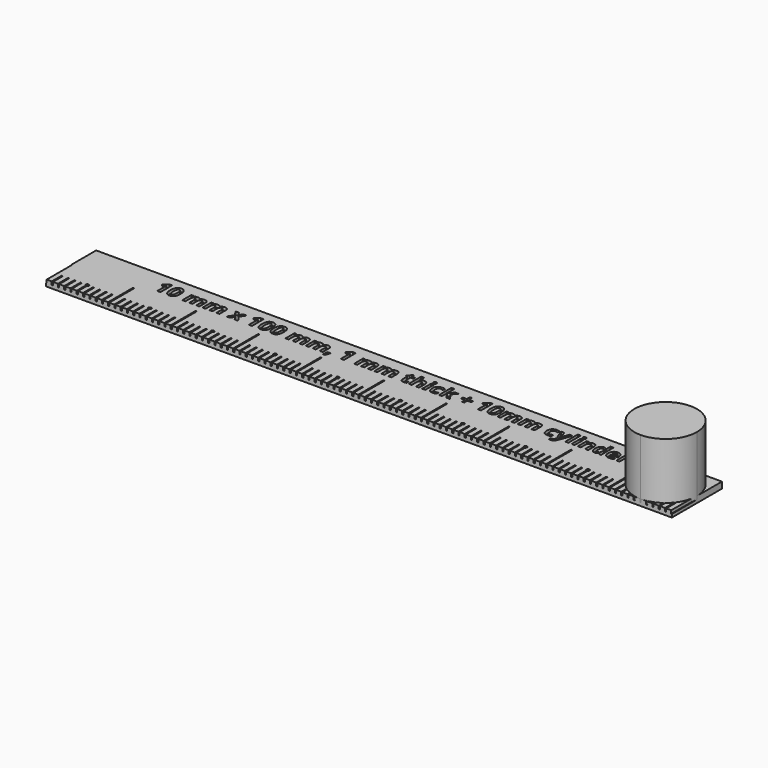
from build123d import *

# Parameters (mm, degrees)
F0_W         = 100
F0_H         = 10
F1_DEPTH     = 0.5
F3_DEPTH     = 0.5
F5_DEPTH     = 10
F6_TEXT_SIZE = 3.2776908483
F7_DEPTH     = 0.5


# Not quite as in the source:
# - Text() gives the source's letters only with a copy of the font that has no kerning and outlines rounded to 1/6400 em; it was checked with that copy


with BuildPart() as f1:
    # F0 (on Top) → F1 (new body)
    with BuildSketch(Plane.XY):
        Rectangle(F0_W, F0_H)
    extrude(amount=F1_DEPTH)

    # F2 (on face) → F3 (join)
    with BuildSketch(Plane.XY.offset(0.5)):
        with BuildLine():
            Line((-49.9, -0.1), (-49.9, -5))
            Line((-49.9, -5), (-49.1, -5))
            Line((-49.1, -5), (-49.1, -3))
            Line((-49.1, -3), (-48.9, -3))
            Line((-48.9, -3), (-48.9, -5))
            Line((-48.9, -5), (-48.1, -5))
            Line((-48.1, -5), (-48.1, -3))
            Line((-48.1, -3), (-47.9, -3))
            Line((-47.9, -3), (-47.9, -5))
            Line((-47.9, -5), (-47.1, -5))
            Line((-47.1, -5), (-47.1, -3))
            Line((-47.1, -3), (-46.9, -3))
            Line((-46.9, -3), (-46.9, -5))
            Line((-46.9, -5), (-46.1, -5))
            Line((-46.1, -5), (-46.1, -3))
            Line((-46.1, -3), (-45.9, -3))
            Line((-45.9, -3), (-45.9, -5))
            Line((-45.9, -5), (-45.1, -5))
            Line((-45.1, -5), (-45.1, -3.2291287847))
            ThreePointArc((-45.1, -3.2291287847), (-45.1369306394, -2.7908349934), (-44.75, -3))
            ThreePointArc((-44.75, -3), (-44.7908349934, -3.1369306394), (-44.9, -3.2291287847))
            Line((-44.9, -3.2291287847), (-44.9, -5))
            Line((-44.9, -5), (-44.1, -5))
            Line((-44.1, -5), (-44.1, -3))
            Line((-44.1, -3), (-43.9, -3))
            Line((-43.9, -3), (-43.9, -5))
            Line((-43.9, -5), (-43.1, -5))
            Line((-43.1, -5), (-43.1, -3))
            Line((-43.1, -3), (-42.9, -3))
            Line((-42.9, -3), (-42.9, -5))
            Line((-42.9, -5), (-42.1, -5))
            Line((-42.1, -5), (-42.1, -3))
            Line((-42.1, -3), (-41.9, -3))
            Line((-41.9, -3), (-41.9, -5))
            Line((-41.9, -5), (-41.1, -5))
            Line((-41.1, -5), (-41.1, -3))
            Line((-41.1, -3), (-40.9, -3))
            Line((-40.9, -3), (-40.9, -5))
            Line((-40.9, -5), (-40.1, -5))
            Line((-40.1, -5), (-40.1, -0.1))
            ThreePointArc((-40.1, -0.1), (-40, 0), (-39.9, -0.1))
            Line((-39.9, -0.1), (-39.9, -5))
            Line((-39.9, -5), (-39.1, -5))
            Line((-39.1, -5), (-39.1, -3))
            Line((-39.1, -3), (-38.9, -3))
            Line((-38.9, -3), (-38.9, -5))
            Line((-38.9, -5), (-38.1, -5))
            Line((-38.1, -5), (-38.1, -3))
            Line((-38.1, -3), (-37.9, -3))
            Line((-37.9, -3), (-37.9, -5))
            Line((-37.9, -5), (-37.1, -5))
            Line((-37.1, -5), (-37.1, -3))
            Line((-37.1, -3), (-36.9, -3))
            Line((-36.9, -3), (-36.9, -5))
            Line((-36.9, -5), (-36.1, -5))
            Line((-36.1, -5), (-36.1, -3))
            Line((-36.1, -3), (-35.9, -3))
            Line((-35.9, -3), (-35.9, -5))
            Line((-35.9, -5), (-35.1, -5))
            Line((-35.1, -5), (-35.1, -3.2291287847))
            ThreePointArc((-35.1, -3.2291287847), (-35.1369306394, -2.7908349934), (-34.75, -3))
            ThreePointArc((-34.75, -3), (-34.7908349934, -3.1369306394), (-34.9, -3.2291287847))
            Line((-34.9, -3.2291287847), (-34.9, -5))
            Line((-34.9, -5), (-34.1, -5))
            Line((-34.1, -5), (-34.1, -3))
            Line((-34.1, -3), (-33.9, -3))
            Line((-33.9, -3), (-33.9, -5))
            Line((-33.9, -5), (-33.1, -5))
            Line((-33.1, -5), (-33.1, -3))
            Line((-33.1, -3), (-32.9, -3))
            Line((-32.9, -3), (-32.9, -5))
            Line((-32.9, -5), (-32.1, -5))
            Line((-32.1, -5), (-32.1, -3))
            Line((-32.1, -3), (-31.9, -3))
            Line((-31.9, -3), (-31.9, -5))
            Line((-31.9, -5), (-31.1, -5))
            Line((-31.1, -5), (-31.1, -3))
            Line((-31.1, -3), (-30.9, -3))
            Line((-30.9, -3), (-30.9, -5))
            Line((-30.9, -5), (-30.1, -5))
            Line((-30.1, -5), (-30.1, -0.1))
            ThreePointArc((-30.1, -0.1), (-30, 0), (-29.9, -0.1))
            Line((-29.9, -0.1), (-29.9, -5))
            Line((-29.9, -5), (-29.1, -5))
            Line((-29.1, -5), (-29.1, -3))
            Line((-29.1, -3), (-28.9, -3))
            Line((-28.9, -3), (-28.9, -5))
            Line((-28.9, -5), (-28.1, -5))
            Line((-28.1, -5), (-28.1, -3))
            Line((-28.1, -3), (-27.9, -3))
            Line((-27.9, -3), (-27.9, -5))
            Line((-27.9, -5), (-27.1, -5))
            Line((-27.1, -5), (-27.1, -3))
            Line((-27.1, -3), (-26.9, -3))
            Line((-26.9, -3), (-26.9, -5))
            Line((-26.9, -5), (-26.1, -5))
            Line((-26.1, -5), (-26.1, -3))
            Line((-26.1, -3), (-25.9, -3))
            Line((-25.9, -3), (-25.9, -5))
            Line((-25.9, -5), (-25.1, -5))
            Line((-25.1, -5), (-25.1, -3.2291287847))
            ThreePointArc((-25.1, -3.2291287847), (-25.1369306394, -2.7908349934), (-24.75, -3))
            ThreePointArc((-24.75, -3), (-24.7908349934, -3.1369306394), (-24.9, -3.2291287847))
            Line((-24.9, -3.2291287847), (-24.9, -5))
            Line((-24.9, -5), (-24.1, -5))
            Line((-24.1, -5), (-24.1, -3))
            Line((-24.1, -3), (-23.9, -3))
            Line((-23.9, -3), (-23.9, -5))
            Line((-23.9, -5), (-23.1, -5))
            Line((-23.1, -5), (-23.1, -3))
            Line((-23.1, -3), (-22.9, -3))
            Line((-22.9, -3), (-22.9, -5))
            Line((-22.9, -5), (-22.1, -5))
            Line((-22.1, -5), (-22.1, -3))
            Line((-22.1, -3), (-21.9, -3))
            Line((-21.9, -3), (-21.9, -5))
            Line((-21.9, -5), (-21.1, -5))
            Line((-21.1, -5), (-21.1, -3))
            Line((-21.1, -3), (-20.9, -3))
            Line((-20.9, -3), (-20.9, -5))
            Line((-20.9, -5), (-20.1, -5))
            Line((-20.1, -5), (-20.1, -0.1))
            ThreePointArc((-20.1, -0.1), (-20, 0), (-19.9, -0.1))
            Line((-19.9, -0.1), (-19.9, -5))
            Line((-19.9, -5), (-19.1, -5))
            Line((-19.1, -5), (-19.1, -3))
            Line((-19.1, -3), (-18.9, -3))
            Line((-18.9, -3), (-18.9, -5))
            Line((-18.9, -5), (-18.1, -5))
            Line((-18.1, -5), (-18.1, -3))
            Line((-18.1, -3), (-17.9, -3))
            Line((-17.9, -3), (-17.9, -5))
            Line((-17.9, -5), (-17.1, -5))
            Line((-17.1, -5), (-17.1, -3))
            Line((-17.1, -3), (-16.9, -3))
            Line((-16.9, -3), (-16.9, -5))
            Line((-16.9, -5), (-16.1, -5))
            Line((-16.1, -5), (-16.1, -3))
            Line((-16.1, -3), (-15.9, -3))
            Line((-15.9, -3), (-15.9, -5))
            Line((-15.9, -5), (-15.1, -5))
            Line((-15.1, -5), (-15.1, -3.2291287847))
            ThreePointArc((-15.1, -3.2291287847), (-15.1369306394, -2.7908349934), (-14.75, -3))
            ThreePointArc((-14.75, -3), (-14.7908349934, -3.1369306394), (-14.9, -3.2291287847))
            Line((-14.9, -3.2291287847), (-14.9, -5))
            Line((-14.9, -5), (-14.1, -5))
            Line((-14.1, -5), (-14.1, -3))
            Line((-14.1, -3), (-13.9, -3))
            Line((-13.9, -3), (-13.9, -5))
            Line((-13.9, -5), (-13.1, -5))
            Line((-13.1, -5), (-13.1, -3))
            Line((-13.1, -3), (-12.9, -3))
            Line((-12.9, -3), (-12.9, -5))
            Line((-12.9, -5), (-12.1, -5))
            Line((-12.1, -5), (-12.1, -3))
            Line((-12.1, -3), (-11.9, -3))
            Line((-11.9, -3), (-11.9, -5))
            Line((-11.9, -5), (-11.1, -5))
            Line((-11.1, -5), (-11.1, -3))
            Line((-11.1, -3), (-10.9, -3))
            Line((-10.9, -3), (-10.9, -5))
            Line((-10.9, -5), (-10.1, -5))
            Line((-10.1, -5), (-10.1, -0.1))
            ThreePointArc((-10.1, -0.1), (-10, 0), (-9.9, -0.1))
            Line((-9.9, -0.1), (-9.9, -5))
            Line((-9.9, -5), (-9.1, -5))
            Line((-9.1, -5), (-9.1, -3))
            Line((-9.1, -3), (-8.9, -3))
            Line((-8.9, -3), (-8.9, -5))
            Line((-8.9, -5), (-8.1, -5))
            Line((-8.1, -5), (-8.1, -3))
            Line((-8.1, -3), (-7.9, -3))
            Line((-7.9, -3), (-7.9, -5))
            Line((-7.9, -5), (-7.1, -5))
            Line((-7.1, -5), (-7.1, -3))
            Line((-7.1, -3), (-6.9, -3))
            Line((-6.9, -3), (-6.9, -5))
            Line((-6.9, -5), (-6.1, -5))
            Line((-6.1, -5), (-6.1, -3))
            Line((-6.1, -3), (-5.9, -3))
            Line((-5.9, -3), (-5.9, -5))
            Line((-5.9, -5), (-5.1, -5))
            Line((-5.1, -5), (-5.1, -3.2291287847))
            ThreePointArc((-5.1, -3.2291287847), (-5.1369306394, -2.7908349934), (-4.75, -3))
            ThreePointArc((-4.75, -3), (-4.7908349934, -3.1369306394), (-4.9, -3.2291287847))
            Line((-4.9, -3.2291287847), (-4.9, -5))
            Line((-4.9, -5), (-4.1, -5))
            Line((-4.1, -5), (-4.1, -3))
            Line((-4.1, -3), (-3.9, -3))
            Line((-3.9, -3), (-3.9, -5))
            Line((-3.9, -5), (-3.1, -5))
            Line((-3.1, -5), (-3.1, -3))
            Line((-3.1, -3), (-2.9, -3))
            Line((-2.9, -3), (-2.9, -5))
            Line((-2.9, -5), (-2.1, -5))
            Line((-2.1, -5), (-2.1, -3))
            Line((-2.1, -3), (-1.9, -3))
            Line((-1.9, -3), (-1.9, -5))
            Line((-1.9, -5), (-1.1, -5))
            Line((-1.1, -5), (-1.1, -3))
            Line((-1.1, -3), (-0.9, -3))
            Line((-0.9, -3), (-0.9, -5))
            Line((-0.9, -5), (-0.1, -5))
            Line((-0.1, -5), (-0.1, -0.1))
            ThreePointArc((-0.1, -0.1), (0, 0), (0.1, -0.1))
            Line((0.1, -0.1), (0.1, -5))
            Line((0.1, -5), (0.9, -5))
            Line((0.9, -5), (0.9, -3))
            Line((0.9, -3), (1.1, -3))
            Line((1.1, -3), (1.1, -5))
            Line((1.1, -5), (1.9, -5))
            Line((1.9, -5), (1.9, -3))
            Line((1.9, -3), (2.1, -3))
            Line((2.1, -3), (2.1, -5))
            Line((2.1, -5), (2.9, -5))
            Line((2.9, -5), (2.9, -3))
            Line((2.9, -3), (3.1, -3))
            Line((3.1, -3), (3.1, -5))
            Line((3.1, -5), (3.9, -5))
            Line((3.9, -5), (3.9, -3))
            Line((3.9, -3), (4.1, -3))
            Line((4.1, -3), (4.1, -5))
            Line((4.1, -5), (4.9, -5))
            Line((4.9, -5), (4.9, -3.2291287847))
            ThreePointArc((4.9, -3.2291287847), (4.8630693606, -2.7908349934), (5.25, -3))
            ThreePointArc((5.25, -3), (5.2091650066, -3.1369306394), (5.1, -3.2291287847))
            Line((5.1, -3.2291287847), (5.1, -5))
            Line((5.1, -5), (5.9, -5))
            Line((5.9, -5), (5.9, -3))
            Line((5.9, -3), (6.1, -3))
            Line((6.1, -3), (6.1, -5))
            Line((6.1, -5), (6.9, -5))
            Line((6.9, -5), (6.9, -3))
            Line((6.9, -3), (7.1, -3))
            Line((7.1, -3), (7.1, -5))
            Line((7.1, -5), (7.9, -5))
            Line((7.9, -5), (7.9, -3))
            Line((7.9, -3), (8.1, -3))
            Line((8.1, -3), (8.1, -5))
            Line((8.1, -5), (8.9, -5))
            Line((8.9, -5), (8.9, -3))
            Line((8.9, -3), (9.1, -3))
            Line((9.1, -3), (9.1, -5))
            Line((9.1, -5), (9.9, -5))
            Line((9.9, -5), (9.9, -0.1))
            ThreePointArc((9.9, -0.1), (10, 0), (10.1, -0.1))
            Line((10.1, -0.1), (10.1, -5))
            Line((10.1, -5), (10.9, -5))
            Line((10.9, -5), (10.9, -3))
            Line((10.9, -3), (11.1, -3))
            Line((11.1, -3), (11.1, -5))
            Line((11.1, -5), (11.9, -5))
            Line((11.9, -5), (11.9, -3))
            Line((11.9, -3), (12.1, -3))
            Line((12.1, -3), (12.1, -5))
            Line((12.1, -5), (12.9, -5))
            Line((12.9, -5), (12.9, -3))
            Line((12.9, -3), (13.1, -3))
            Line((13.1, -3), (13.1, -5))
            Line((13.1, -5), (13.9, -5))
            Line((13.9, -5), (13.9, -3))
            Line((13.9, -3), (14.1, -3))
            Line((14.1, -3), (14.1, -5))
            Line((14.1, -5), (14.9, -5))
            Line((14.9, -5), (14.9, -3.2291287847))
            ThreePointArc((14.9, -3.2291287847), (14.8630693606, -2.7908349934), (15.25, -3))
            ThreePointArc((15.25, -3), (15.2091650066, -3.1369306394), (15.1, -3.2291287847))
            Line((15.1, -3.2291287847), (15.1, -5))
            Line((15.1, -5), (15.9, -5))
            Line((15.9, -5), (15.9, -3))
            Line((15.9, -3), (16.1, -3))
            Line((16.1, -3), (16.1, -5))
            Line((16.1, -5), (16.9, -5))
            Line((16.9, -5), (16.9, -3))
            Line((16.9, -3), (17.1, -3))
            Line((17.1, -3), (17.1, -5))
            Line((17.1, -5), (17.9, -5))
            Line((17.9, -5), (17.9, -3))
            Line((17.9, -3), (18.1, -3))
            Line((18.1, -3), (18.1, -5))
            Line((18.1, -5), (18.9, -5))
            Line((18.9, -5), (18.9, -3))
            Line((18.9, -3), (19.1, -3))
            Line((19.1, -3), (19.1, -5))
            Line((19.1, -5), (19.9, -5))
            Line((19.9, -5), (19.9, -0.1))
            ThreePointArc((19.9, -0.1), (20, 0), (20.1, -0.1))
            Line((20.1, -0.1), (20.1, -5))
            Line((20.1, -5), (20.9, -5))
            Line((20.9, -5), (20.9, -3))
            Line((20.9, -3), (21.1, -3))
            Line((21.1, -3), (21.1, -5))
            Line((21.1, -5), (21.9, -5))
            Line((21.9, -5), (21.9, -3))
            Line((21.9, -3), (22.1, -3))
            Line((22.1, -3), (22.1, -5))
            Line((22.1, -5), (22.9, -5))
            Line((22.9, -5), (22.9, -3))
            Line((22.9, -3), (23.1, -3))
            Line((23.1, -3), (23.1, -5))
            Line((23.1, -5), (23.9, -5))
            Line((23.9, -5), (23.9, -3))
            Line((23.9, -3), (24.1, -3))
            Line((24.1, -3), (24.1, -5))
            Line((24.1, -5), (24.9, -5))
            Line((24.9, -5), (24.9, -3.2291287847))
            ThreePointArc((24.9, -3.2291287847), (24.8630693606, -2.7908349934), (25.25, -3))
            ThreePointArc((25.25, -3), (25.2091650066, -3.1369306394), (25.1, -3.2291287847))
            Line((25.1, -3.2291287847), (25.1, -5))
            Line((25.1, -5), (25.9, -5))
            Line((25.9, -5), (25.9, -3))
            Line((25.9, -3), (26.1, -3))
            Line((26.1, -3), (26.1, -5))
            Line((26.1, -5), (26.9, -5))
            Line((26.9, -5), (26.9, -3))
            Line((26.9, -3), (27.1, -3))
            Line((27.1, -3), (27.1, -5))
            Line((27.1, -5), (27.9, -5))
            Line((27.9, -5), (27.9, -3))
            Line((27.9, -3), (28.1, -3))
            Line((28.1, -3), (28.1, -5))
            Line((28.1, -5), (28.9, -5))
            Line((28.9, -5), (28.9, -3))
            Line((28.9, -3), (29.1, -3))
            Line((29.1, -3), (29.1, -5))
            Line((29.1, -5), (29.9, -5))
            Line((29.9, -5), (29.9, -0.1))
            ThreePointArc((29.9, -0.1), (30, 0), (30.1, -0.1))
            Line((30.1, -0.1), (30.1, -5))
            Line((30.1, -5), (30.9, -5))
            Line((30.9, -5), (30.9, -3))
            Line((30.9, -3), (31.1, -3))
            Line((31.1, -3), (31.1, -5))
            Line((31.1, -5), (31.9, -5))
            Line((31.9, -5), (31.9, -3))
            Line((31.9, -3), (32.1, -3))
            Line((32.1, -3), (32.1, -5))
            Line((32.1, -5), (32.9, -5))
            Line((32.9, -5), (32.9, -3))
            Line((32.9, -3), (33.1, -3))
            Line((33.1, -3), (33.1, -5))
            Line((33.1, -5), (33.9, -5))
            Line((33.9, -5), (33.9, -3))
            Line((33.9, -3), (34.1, -3))
            Line((34.1, -3), (34.1, -5))
            Line((34.1, -5), (34.9, -5))
            Line((34.9, -5), (34.9, -3.2291287847))
            ThreePointArc((34.9, -3.2291287847), (34.8630693606, -2.7908349934), (35.25, -3))
            ThreePointArc((35.25, -3), (35.2091650066, -3.1369306394), (35.1, -3.2291287847))
            Line((35.1, -3.2291287847), (35.1, -5))
            Line((35.1, -5), (35.9, -5))
            Line((35.9, -5), (35.9, -3))
            Line((35.9, -3), (36.1, -3))
            Line((36.1, -3), (36.1, -5))
            Line((36.1, -5), (36.9, -5))
            Line((36.9, -5), (36.9, -3))
            Line((36.9, -3), (37.1, -3))
            Line((37.1, -3), (37.1, -5))
            Line((37.1, -5), (37.9, -5))
            Line((37.9, -5), (37.9, -3))
            Line((37.9, -3), (38.1, -3))
            Line((38.1, -3), (38.1, -5))
            Line((38.1, -5), (38.9, -5))
            Line((38.9, -5), (38.9, -3))
            Line((38.9, -3), (39.1, -3))
            Line((39.1, -3), (39.1, -5))
            Line((39.1, -5), (39.9, -5))
            Line((39.9, -5), (39.9, -0.1))
            ThreePointArc((39.9, -0.1), (40, 0), (40.1, -0.1))
            Line((40.1, -0.1), (40.1, -5))
            Line((40.1, -5), (40.9, -5))
            Line((40.9, -5), (40.9, -3))
            Line((40.9, -3), (41.1, -3))
            Line((41.1, -3), (41.1, -5))
            Line((41.1, -5), (41.9, -5))
            Line((41.9, -5), (41.9, -3))
            Line((41.9, -3), (42.1, -3))
            Line((42.1, -3), (42.1, -5))
            Line((42.1, -5), (42.9, -5))
            Line((42.9, -5), (42.9, -3))
            Line((42.9, -3), (43.1, -3))
            Line((43.1, -3), (43.1, -5))
            Line((43.1, -5), (43.9, -5))
            Line((43.9, -5), (43.9, -3))
            Line((43.9, -3), (44.1, -3))
            Line((44.1, -3), (44.1, -5))
            Line((44.1, -5), (44.9, -5))
            Line((44.9, -5), (44.9, -3.2291287847))
            ThreePointArc((44.9, -3.2291287847), (44.8630693606, -2.7908349934), (45.25, -3))
            ThreePointArc((45.25, -3), (45.2091650066, -3.1369306394), (45.1, -3.2291287847))
            Line((45.1, -3.2291287847), (45.1, -5))
            Line((45.1, -5), (45.9, -5))
            Line((45.9, -5), (45.9, -3))
            Line((45.9, -3), (46.1, -3))
            Line((46.1, -3), (46.1, -5))
            Line((46.1, -5), (46.9, -5))
            Line((46.9, -5), (46.9, -3))
            Line((46.9, -3), (47.1, -3))
            Line((47.1, -3), (47.1, -5))
            Line((47.1, -5), (47.9, -5))
            Line((47.9, -5), (47.9, -3))
            Line((47.9, -3), (48.1, -3))
            Line((48.1, -3), (48.1, -5))
            Line((48.1, -5), (48.9, -5))
            Line((48.9, -5), (48.9, -3))
            Line((48.9, -3), (49.1, -3))
            Line((49.1, -3), (49.1, -5))
            Line((49.1, -5), (49.9, -5))
            Line((49.9, -5), (49.9, -0.1))
            ThreePointArc((49.9, -0.1), (49.9292893219, -0.0292893219), (50, 0))
            Line((50, 0), (50, 5))
            Line((50, 5), (-50, 5))
            Line((-50, 5), (-50, 0))
            ThreePointArc((-50, 0), (-49.9292893219, -0.0292893219), (-49.9, -0.1))
        make_face()
    extrude(amount=F3_DEPTH)

    # F4 (on face) → F5 (join)
    with BuildSketch(Plane(origin=(0, 0, 0), x_dir=(1, 0, 0), z_dir=(0, 0, -1))):
        with BuildLine():
            ThreePointArc((45, -5), (48.5355339059, -3.5355339059), (50, 0))
            ThreePointArc((50, 0), (48.5355339059, 3.5355339059), (45, 5))
            ThreePointArc((45, 5), (40, 0), (45, -5))
        make_face()
    extrude(amount=-F5_DEPTH)

    # F6 (on face) → F7 (cut)
    with BuildSketch(Plane.XY.offset(1)):
        with Locations((-38.0485344649, 1.2145340443)):
            Text('10 mm x 100 mm, 1 mm thick + 10mm cylinder', F6_TEXT_SIZE, font='Open Sans', font_style=FontStyle.BOLD, text_align=(TextAlign.LEFT, TextAlign.BOTTOM))
    extrude(amount=-F7_DEPTH, mode=Mode.SUBTRACT)


solid = f1.part
